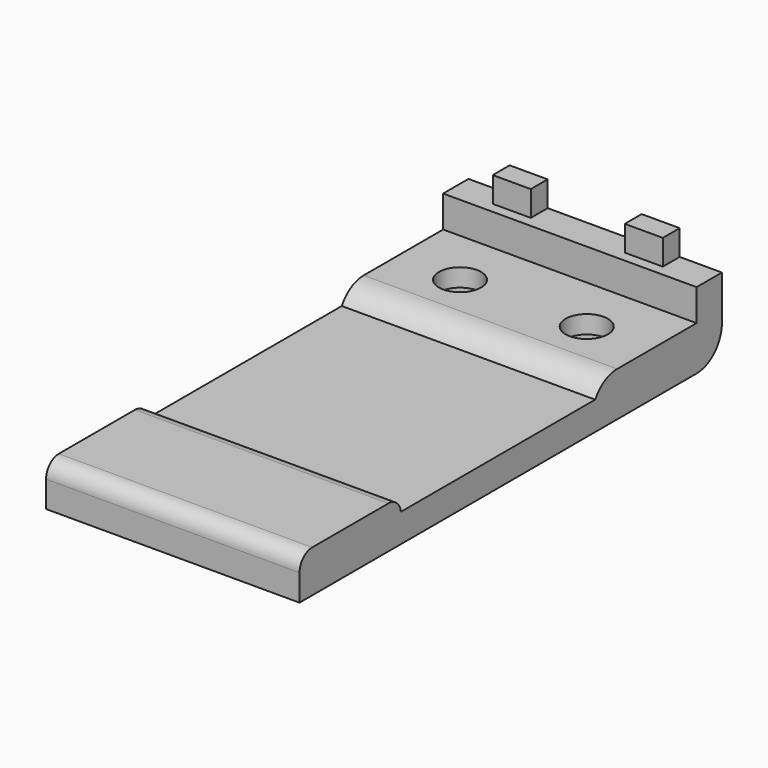
from build123d import *

# Parameters (mm, degrees)
F0_W        = 24
F0_H        = 12
F0_H_2      = 23
F0_R        = 4.3
F0_H_3      = 3
F1_DEPTH    = 2.7
F0_R_2      = 2
F2_DEPTH    = 4.2
F3_DEPTH    = 2.5
F4_DEPTH    = 7.2
F5_W        = 3.6
F5_H        = 2
F6_DEPTH    = 2.4
F7_T1_DEPTH = 39
F7_T3_DEPTH = 36.9903810568
F8_DEPTH    = 4
F9_T1_DEPTH = 31.4330343737
F9_T3_DEPTH = 31.5


# Not quite as in the source:
# - a fillet or chamfer that OpenCascade refuses, or shapes differently, is made with other operations: its cross-section is extruded or revolved along the edge and cut away or added


with BuildPart() as f1:
    # F0 (on Top) → F1 (new body)
    with BuildSketch(Plane.XY):
        with Locations((12, -44)):
            Rectangle(F0_W, F0_H)
        with Locations((12, -26.5)):
            Rectangle(F0_W, F0_H_2)
        with Locations((12, -9)):
            Rectangle(F0_W, F0_H)
        with Locations((6, -8.5)):
            Circle(F0_R, mode=Mode.SUBTRACT)
        with Locations((18, -8.5)):
            Circle(F0_R, mode=Mode.SUBTRACT)
        with Locations((12, -1.5)):
            Rectangle(F0_W, F0_H_3)
    extrude(amount=F1_DEPTH)

    # F0 (on Top) → F2 (join)
    with BuildSketch(Plane.XY):
        with Locations((12, -1.5)):
            Rectangle(F0_W, F0_H_3)
        with Locations((12, -9)):
            Rectangle(F0_W, F0_H)
        with Locations((6, -8.5)):
            Circle(F0_R, mode=Mode.SUBTRACT)
        with Locations((18, -8.5)):
            Circle(F0_R, mode=Mode.SUBTRACT)
        with Locations((6, -8.5)):
            Circle(F0_R)
        with Locations((6, -8.5)):
            Circle(F0_R_2, mode=Mode.SUBTRACT)
        with Locations((18, -8.5)):
            Circle(F0_R)
        with Locations((18, -8.5)):
            Circle(F0_R_2, mode=Mode.SUBTRACT)
    extrude(amount=F2_DEPTH)

    # F0 (on Top) → F3 (cut)
    with BuildSketch(Plane.XY):
        with Locations((6, -8.5)):
            Circle(F0_R)
        with Locations((6, -8.5)):
            Circle(F0_R_2, mode=Mode.SUBTRACT)
        with Locations((18, -8.5)):
            Circle(F0_R)
        with Locations((18, -8.5)):
            Circle(F0_R_2, mode=Mode.SUBTRACT)
    extrude(amount=F3_DEPTH, mode=Mode.SUBTRACT)

    # F0 (on Top) → F4 (join)
    with BuildSketch(Plane.XY):
        with Locations((12, -1.5)):
            Rectangle(F0_W, F0_H_3)
    extrude(amount=F4_DEPTH)

    # F5 (on face) → F6 (join)
    with BuildSketch(Plane.XY.offset(7.2)):
        with Locations((5.7, -1)):
            Rectangle(F5_W, F5_H)
        with Locations((18.2, -1)):
            Rectangle(F5_W, F5_H)
    extrude(amount=F6_DEPTH)

    # F7: fillet of radius 3 on 2 edges, made by hand

    # F7_s2 → F7_t1 (cut)
    with BuildSketch(Plane.YZ.offset(-7.5)):
        with BuildLine():
            ThreePointArc((-3, 0), (-0.8786796564, 0.8786796564), (0, 3))
            Line((0, 3), (0, 0))
            Line((0, 0), (-3, 0))
        make_face()
    extrude(amount=F7_T1_DEPTH, mode=Mode.SUBTRACT)

    # F7_s4 → F7_t3 (cut)
    with BuildSketch(Plane.YZ.offset(-6.4951905284)):
        with BuildLine():
            ThreePointArc((-12.4019237886, 4.2), (-13.9019237886, 3.7980762114), (-15, 2.7))
            Line((-15, 2.7), (-15, 4.2))
            Line((-15, 4.2), (-12.4019237886, 4.2))
        make_face()
    extrude(amount=F7_T3_DEPTH, mode=Mode.SUBTRACT)

    # F0 (on Top) → F8 (join)
    with BuildSketch(Plane.XY):
        with Locations((12, -44)):
            Rectangle(F0_W, F0_H)
    extrude(amount=F8_DEPTH)

    # F9: fillet of radius 1.5 on 2 edges, made by hand

    # F9_s2 → F9_t1 (cut)
    with BuildSketch(Plane.YZ.offset(-3.7165171868)):
        with BuildLine():
            ThreePointArc((-38, 2.7), (-38.4991859918, 3.6291589791), (-39.4866068747, 4))
            Line((-39.4866068747, 4), (-38, 4))
            Line((-38, 4), (-38, 2.7))
        make_face()
    extrude(amount=F9_T1_DEPTH, mode=Mode.SUBTRACT)

    # F9_s4 → F9_t3 (cut)
    with BuildSketch(Plane.YZ.offset(-3.75)):
        with BuildLine():
            ThreePointArc((-50, 2.5), (-49.5606601718, 3.5606601718), (-48.5, 4))
            Line((-48.5, 4), (-50, 4))
            Line((-50, 4), (-50, 2.5))
        make_face()
    extrude(amount=F9_T3_DEPTH, mode=Mode.SUBTRACT)


solid = f1.part
